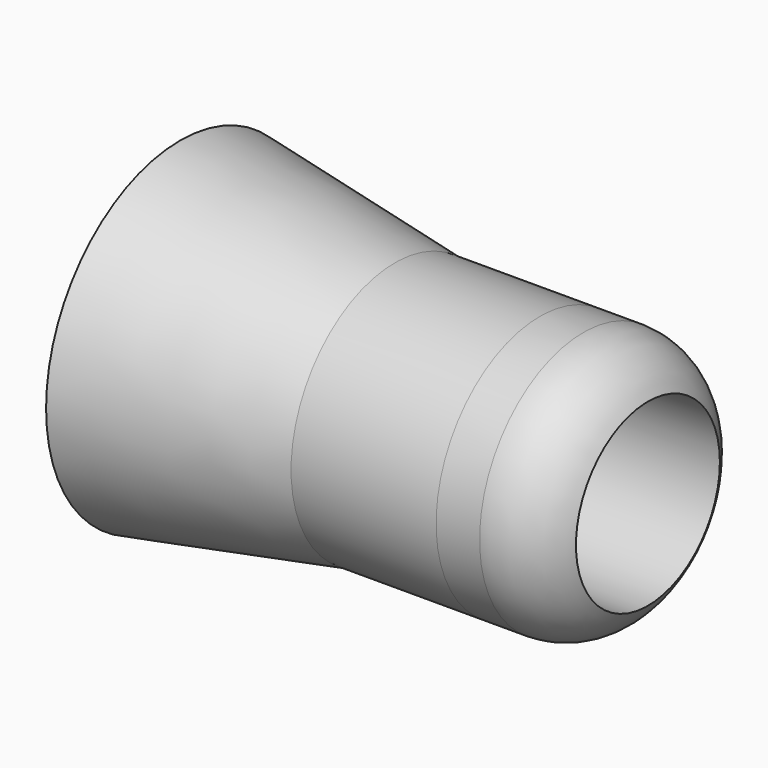
from build123d import *

# Parameters (mm, degrees)
F0_R        = 12.4431552
F0_R_2      = 9.1690063
F1_DEPTH    = 12.7
F0_R_3      = 6.35
F2_DEPTH    = 20.32
F3_S5_R     = 9.1690063
F3_T6_DEPTH = 24


# Not quite as in the source:
# - a fillet or chamfer that OpenCascade refuses, or shapes differently, is made with other operations: its cross-section is extruded or revolved along the edge and cut away or added


with BuildPart() as f1:
    # F0 (on Right) → F1 (new body, symmetric)
    with BuildSketch(Plane.YZ):
        Circle(F0_R)
        Circle(F0_R_2, mode=Mode.SUBTRACT)
    extrude(amount=F1_DEPTH, both=True)

    # F0 (on Right) → F2 (join)
    with BuildSketch(Plane.YZ):
        Circle(F0_R_2)
        Circle(F0_R_3, mode=Mode.SUBTRACT)
    extrude(amount=F2_DEPTH)

    # F3: chamfer of 5.08 x 28.8101116437 on 1 edges, made by hand


with BuildPart() as f3_tool2:
    # F3_s3 → F3_t4 (revolve)
    with BuildSketch(Plane.XY):
        Polygon((-16.1101116437, 12.4431552), (12.7, 7.3631552), (12.7, 12.4431552), align=None)
    revolve(axis=Axis((12.7, 0, 0), (1, 0, 0)))

    # F3_s5 → F3_t6 (cut, symmetric)
    with BuildSketch(Plane.YZ.offset(-1.7)):
        Circle(F3_S5_R)
    extrude(amount=F3_T6_DEPTH, both=True, mode=Mode.SUBTRACT)


with BuildPart() as f1_1:
    add(f1.part)

    # F3_t1: cut F3_tool2
    add(f3_tool2.part, mode=Mode.SUBTRACT)

    # F4: fillet of radius 5.08 on 1 edges, made by hand

    # F4_s1 → F4_t2 (revolve, cut)
    with BuildSketch(Plane.XY):
        with BuildLine():
            ThreePointArc((15.7709003651, 9.1690063), (18.44676957, 8.4071220926), (20.32, 6.35))
            Line((20.32, 6.35), (20.32, 9.1690063))
            Line((20.32, 9.1690063), (15.7709003651, 9.1690063))
        make_face()
    revolve(axis=Axis((20.32, 0, 0), (1, 0, 0)), mode=Mode.SUBTRACT)


solid = f1_1.part
